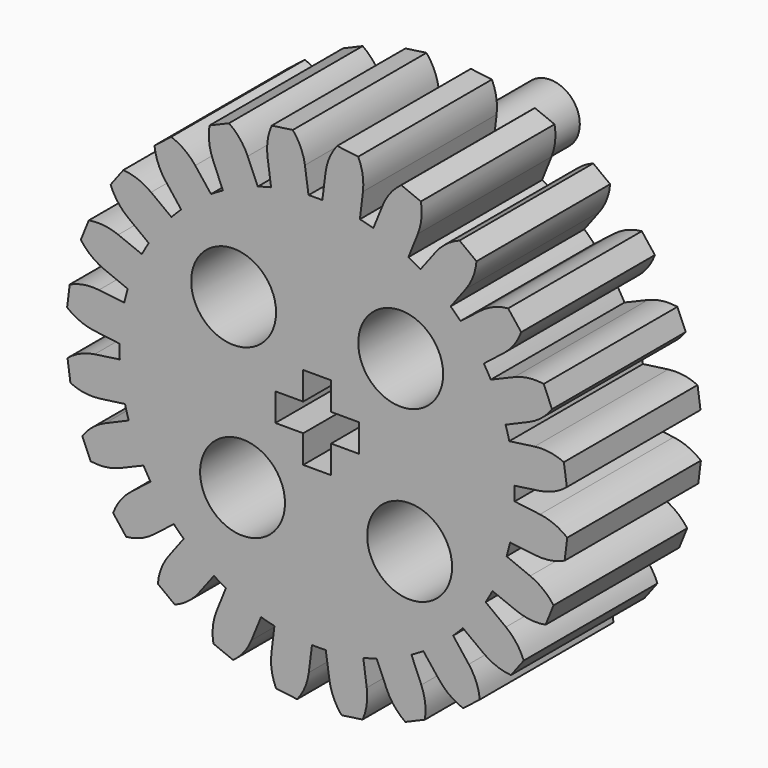
from build123d import *

# Parameters (mm, degrees)
F2_R            = 9.46
F2_R_2          = 2.0320626532
F3_DEPTH        = 8
F4_DEPTH        = 8
F4_COPIES_COUNT = 24
F6_DEPTH        = 25.4
F7_R            = 1.4171024219
F8_DEPTH        = 6.35


# Not quite as in the source:
# - a pattern or mirror of a feature is missing from the dataset's text; its kind, count and spacing are read off the source's solid


with BuildPart() as f3:
    # F2 (on Front) → F3 (new body)
    with BuildSketch(Plane.XZ):
        Circle(F2_R)
        with Locations((-3.5724579239, -3.8998227125)):
            Circle(F2_R_2, mode=Mode.SUBTRACT)
        with Locations((4.4270495434, -3.9885936614)):
            Circle(F2_R_2, mode=Mode.SUBTRACT)
        with Locations((-4, 4)):
            Circle(F2_R_2, mode=Mode.SUBTRACT)
        with Locations((4, 4)):
            Circle(F2_R_2, mode=Mode.SUBTRACT)
    extrude(amount=F3_DEPTH)

    # F0 (on Front) → F4 (join, through all)
    with BuildSketch(Plane.XZ):
        with BuildLine():
            Line((1.9666390983, 11.8486449874), (0.9582122082, 11.9724642403))
            ThreePointArc((0.9582122082, 11.9724642403), (0.5880905232, 11.3584114534), (0.4006877554, 10.66636298))
            Line((0.4006877554, 10.66636298), (0.2481307522, 9.4567452715))
            ThreePointArc((0.2481307522, 9.4567452715), (1.1528778692, 9.3894873459), (2.0470214954, 9.2358704515))
            Line((2.0470214954, 9.2358704515), (2.1916287959, 10.4464642598))
            ThreePointArc((2.1916287959, 10.4464642598), (2.1772140976, 11.1632922692), (1.9666390983, 11.8486449874))
        make_face()
    f4 = extrude(amount=F4_DEPTH)

    # F4_copies: F4 ×24 about axis
    f4_copies_axis = Axis((0, 0, 0), (0, 1, 0))
    for i in range(1, F4_COPIES_COUNT):
        add(f4.rotate(f4_copies_axis, i * 360 / F4_COPIES_COUNT))

    # F5 (on Front) → F6 (cut)
    with BuildSketch(Plane.XZ):
        Polygon((0.666306405, 0.666306405), (0.666306405, 1.9996397384), (-0.0003602616, 1.9996397384), (-0.6670269283, 1.9996397384), (-0.6670269283, 0.666306405), (-2.0003602616, 0.666306405), (-2.0003602616, -0.0003602616), (-2.0003602616, -0.6670269283), (-0.6670269283, -0.6670269283), (-0.6670269283, -2.0003602616), (-0.0003602616, -2.0003602616), (0.666306405, -2.0003602616), (0.666306405, -0.6670269283), (1.9996397384, -0.6670269283), (1.9996397384, -0.0003602616), (1.9996397384, 0.666306405), align=None)
    extrude(amount=F6_DEPTH, mode=Mode.SUBTRACT)

    # F7 (on Front) → F8 (join)
    with BuildSketch(Plane.XZ):
        with Locations((-0.3211766889, 7.1003306657)):
            Circle(F7_R)
    extrude(amount=-F8_DEPTH)


solid = f3.part
